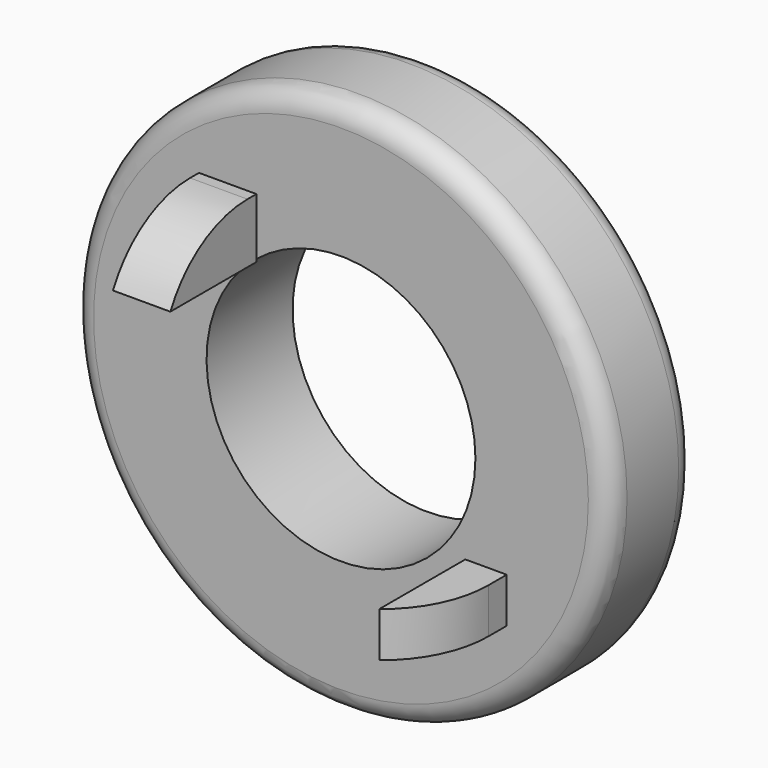
from build123d import *

# Parameters (mm, degrees)
F0_R        = 63.5
F0_R_2      = 31.75
F1_DEPTH    = 25.4
F2_R        = 5.08
F3_R        = 5.08
F6_W        = 9.770580698
F6_H        = 10.6324088763
F6_W_2      = 13.55634837
F6_H_2      = 14.134524271
F7_DEPTH    = 25.4
F8_T1_DEPTH = 127.3817691468
F9_T1_DEPTH = 110.742504806


# Not quite as in the source:
# - a fillet or chamfer that OpenCascade refuses, or shapes differently, is made with other operations: its cross-section is extruded or revolved along the edge and cut away or added
# - the program builds the solid bodies; features that only make, move or delete a surface that nothing else refers to are left out


with BuildPart() as f1:
    # F0 (on Front) → F1 (new body)
    with BuildSketch(Plane.XZ):
        Circle(F0_R)
        Circle(F0_R_2, mode=Mode.SUBTRACT)
    extrude(amount=F1_DEPTH)

    # F2
    f2_edges = [f1.edges().sort_by_distance(p)[0] for p in [
        (-63.5, -25.4, 0),
    ]]
    fillet(f2_edges, radius=F2_R)

    # F3
    f3_edges = [f1.edges().sort_by_distance(p)[0] for p in [
        (-63.5, 0, 0),
    ]]
    fillet(f3_edges, radius=F3_R)

    # F6 (on face) → F7 (join)
    with BuildSketch(Plane.XZ.offset(25.4)):
        with Locations((34.2497480866, -27.0734353661)):
            Rectangle(F6_W, F6_H)
        with Locations((-26.7572421814, 31.0905136006)):
            Rectangle(F6_W_2, F6_H_2)
    extrude(amount=F7_DEPTH)

    # F8: fillet of radius 25.4 on 1 edges, made by hand

    # F8_s2 → F8_t1 (cut)
    with BuildSketch(Plane.YZ.offset(-90.4481267548)):
        with BuildLine():
            ThreePointArc((-28.0349158446, 38.1577757361), (-41.4329925067, 34.3367363635), (-50.8, 24.0232514651))
            Line((-50.8, 24.0232514651), (-50.8, 38.1577757361))
            Line((-50.8, 38.1577757361), (-28.0349158446, 38.1577757361))
        make_face()
    extrude(amount=F8_T1_DEPTH, mode=Mode.SUBTRACT)

    # F9: fillet of radius 25.4 on 1 edges, made by hand

    # F9_s2 → F9_t1 (cut)
    with BuildSketch(Plane.XY.offset(-82.4446877691)):
        with BuildLine():
            ThreePointArc((39.1350384356, -30.777980814), (36.5620755875, -41.9173872105), (29.3644577376, -50.8))
            Line((29.3644577376, -50.8), (39.1350384356, -50.8))
            Line((39.1350384356, -50.8), (39.1350384356, -30.777980814))
        make_face()
    extrude(amount=F9_T1_DEPTH, mode=Mode.SUBTRACT)


solid = f1.part
